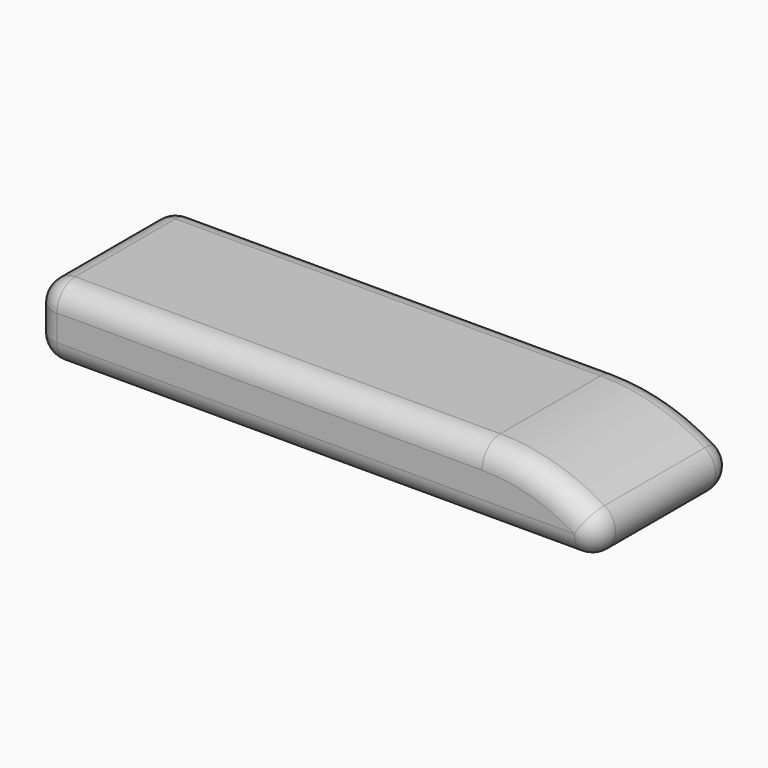
from build123d import *

# Parameters (mm, degrees)
F1_DEPTH     = 38.1
F2_R         = 5.08
F3_F1_R      = 5.08
F3_T2_DEPTH  = 94.7599984092
F3_T4_DEPTH  = 115.3407412507
F3_S8_W      = 5.1816
F3_S8_H      = 5.1816
F3_T9_DEPTH  = 5.1816
F3_S14_W     = 5.1816
F3_S14_H     = 5.1816
F3_T15_DEPTH = 5.1816
F3_T19_ANGLE = 31.4774656297
F3_T21_ANGLE = 148.5225343703
F3_T22_DEPTH = 94.7599984092
F3_T24_DEPTH = 115.3407412507
F3_S28_W     = 5.1816
F3_S28_H     = 5.1816
F3_T29_DEPTH = 5.1816
F3_S34_W     = 5.1816
F3_S34_H     = 5.1816
F3_T35_DEPTH = 5.1816
F3_T39_ANGLE = 31.4774656297
F3_T41_ANGLE = 148.5225343703


# Not quite as in the source:
# - a fillet or chamfer that OpenCascade refuses, or shapes differently, is made with other operations: its cross-section is extruded or revolved along the edge and cut away or added


with BuildPart() as f1:
    # F0 (on Front) → F1 (new body)
    with BuildSketch(Plane.XZ):
        with BuildLine():
            Line((9.9600013345, 7.7700004913), (-89.8799970746, 7.7700004913))
            Line((-89.8799970746, 7.7700004913), (-89.8799970746, -8.1900004297))
            Line((-89.8799970746, -8.1900004297), (44.0999977291, -8.1900004297))
            ThreePointArc((44.0999977291, -8.1900004297), (28.8031763803, 3.5829980082), (9.9600013345, 7.7700004913))
        make_face()
    extrude(amount=F1_DEPTH)

    # F2
    f2_edges = [f1.edges().sort_by_distance(p)[0] for p in [
        (-89.879997, -19.05, -8.19),
        (-89.879997, 0, -0.21),
        (-89.879997, -19.05, 7.77),
        (-89.879997, -38.1, -0.21),
    ]]
    fillet(f2_edges, radius=F2_R)

    # F3: fillet of radius 5.08 on 12 edges, made by hand

    # F3_f1
    f3_f1_edges = [f1.edges().sort_by_distance(p)[0] for p in [
        (44.0999977291, -19.05, -8.1900004297),
    ]]
    fillet(f3_f1_edges, radius=F3_F1_R)

    # F3_s3 → F3_t2 (cut)
    with BuildSketch(Plane.YZ.offset(-84.7999970746)):
        with BuildLine():
            ThreePointArc((0, 2.6900004913), (-1.4878975516, 6.2821029397), (-5.08, 7.7700004913))
            Line((-5.08, 7.7700004913), (-5.08, 7.8716004913))
            Line((-5.08, 7.8716004913), (0.1016, 7.8716004913))
            Line((0.1016, 7.8716004913), (0.1016, 2.6900004913))
            Line((0.1016, 2.6900004913), (0, 2.6900004913))
        make_face()
    extrude(amount=F3_T2_DEPTH, mode=Mode.SUBTRACT)

    # F3_s5 → F3_t4 (cut)
    with BuildSketch(Plane.YZ.offset(-84.7999970746)):
        with BuildLine():
            ThreePointArc((0, -3.1100004297), (-1.4878975516, -6.7021028782), (-5.08, -8.1900004297))
            Line((-5.08, -8.1900004297), (-5.08, -8.2916004297))
            Line((-5.08, -8.2916004297), (0.1016, -8.2916004297))
            Line((0.1016, -8.2916004297), (0.1016, -3.1100004297))
            Line((0.1016, -3.1100004297), (0, -3.1100004297))
        make_face()
    extrude(amount=F3_T4_DEPTH, mode=Mode.SUBTRACT)


with BuildPart() as f3_tool7:
    # F3_s8 → F3_t9 (new body)
    with BuildSketch(Plane.XZ.offset(5.08)):
        with Locations((-87.3907970746, 5.2808004913)):
            Rectangle(F3_S8_W, F3_S8_H)
    extrude(amount=-F3_T9_DEPTH)

    # F3_s10 → F3_t11 (revolve, cut)
    with BuildSketch(Plane(origin=(-84.7999970746, -5.08, 2.6900004913), x_dir=(0.7071067812, 0, -0.7071067812), z_dir=(0.7071067812, 0, 0.7071067812))):
        with BuildLine():
            ThreePointArc((0, -5.08), (5.08, 0), (0, 5.08))
            Line((0, 5.08), (0, -5.08))
        make_face()
    revolve(axis=Axis((-84.7999970746, -5.08, 2.6900004913), (0, 1, 0)), mode=Mode.SUBTRACT)


with BuildPart() as f1_1:
    add(f1.part)

    # F3_t6: cut F3_tool7
    add(f3_tool7.part, mode=Mode.SUBTRACT)


with BuildPart() as f3_tool13:
    # F3_s14 → F3_t15 (new body)
    with BuildSketch(Plane.XZ.offset(5.08)):
        with Locations((-87.3907970746, -5.7008004297)):
            Rectangle(F3_S14_W, F3_S14_H)
    extrude(amount=-F3_T15_DEPTH)

    # F3_s16 → F3_t17 (revolve, cut)
    with BuildSketch(Plane(origin=(-84.7999970746, -5.08, -3.1100004297), x_dir=(0.7071067812, 0, 0.7071067812), z_dir=(-0.7071067812, 0, 0.7071067812))):
        with BuildLine():
            ThreePointArc((0, -5.08), (5.08, 0), (0, 5.08))
            Line((0, 5.08), (0, -5.08))
        make_face()
    revolve(axis=Axis((-84.7999970746, -5.08, -3.1100004297), (0, 1, 0)), mode=Mode.SUBTRACT)


with BuildPart() as f1_2:
    add(f1_1.part)

    # F3_t12: cut F3_tool13
    add(f3_tool13.part, mode=Mode.SUBTRACT)

    # F3_s18 → F3_t19 (revolve, cut)
    with BuildSketch(Plane(origin=(23.5986358548, 0, -14.4484990421), x_dir=(0, 1, 0), z_dir=(0.8528455965, 0, -0.5221631818))):
        with BuildLine():
            ThreePointArc((0, 13.2949019826), (-1.4878975516, 16.887004431), (-5.08, 18.3749019826))
            Line((-5.08, 18.3749019826), (-5.08, 18.4765019826))
            Line((-5.08, 18.4765019826), (0.1016, 18.4765019826))
            Line((0.1016, 18.4765019826), (0.1016, 13.2949019826))
            Line((0.1016, 13.2949019826), (0, 13.2949019826))
        make_face()
    revolve(axis=Axis((9.9600013345, 0, -36.7243886458), (0, -1, 0)), revolution_arc=F3_T19_ANGLE, mode=Mode.SUBTRACT)

    # F3_s20 → F3_t21 (revolve, cut)
    with BuildSketch(Plane(origin=(23.5986358548, 0, -14.4484990421), x_dir=(0, 1, 0), z_dir=(-0.8528455965, 0, 0.5221631818))):
        with BuildLine():
            ThreePointArc((0, -13.2949019826), (-1.4878975516, -16.887004431), (-5.08, -18.3749019826))
            Line((-5.08, -18.3749019826), (-5.08, -18.4765019826))
            Line((-5.08, -18.4765019826), (0.1016, -18.4765019826))
            Line((0.1016, -18.4765019826), (0.1016, -13.2949019826))
            Line((0.1016, -13.2949019826), (0, -13.2949019826))
        make_face()
    revolve(axis=Axis((30.5407441761, 0, -3.1100004297), (0, 1, 0)), revolution_arc=F3_T21_ANGLE, mode=Mode.SUBTRACT)

    # F3_s23 → F3_t22 (cut)
    with BuildSketch(Plane.YZ.offset(-84.7999970746)):
        with BuildLine():
            ThreePointArc((-33.02, 7.7700004913), (-36.6121024484, 6.2821029397), (-38.1, 2.6900004913))
            Line((-38.1, 2.6900004913), (-38.2016, 2.6900004913))
            Line((-38.2016, 2.6900004913), (-38.2016, 7.8716004913))
            Line((-38.2016, 7.8716004913), (-33.02, 7.8716004913))
            Line((-33.02, 7.8716004913), (-33.02, 7.7700004913))
        make_face()
    extrude(amount=F3_T22_DEPTH, mode=Mode.SUBTRACT)

    # F3_s25 → F3_t24 (cut)
    with BuildSketch(Plane.YZ.offset(-84.7999970746)):
        with BuildLine():
            ThreePointArc((-33.02, -8.1900004297), (-36.6121024484, -6.7021028782), (-38.1, -3.1100004297))
            Line((-38.1, -3.1100004297), (-38.2016, -3.1100004297))
            Line((-38.2016, -3.1100004297), (-38.2016, -8.2916004297))
            Line((-38.2016, -8.2916004297), (-33.02, -8.2916004297))
            Line((-33.02, -8.2916004297), (-33.02, -8.1900004297))
        make_face()
    extrude(amount=F3_T24_DEPTH, mode=Mode.SUBTRACT)


with BuildPart() as f3_tool27:
    # F3_s28 → F3_t29 (new body)
    with BuildSketch(Plane.XY.offset(2.6900004913)):
        with Locations((-87.3907970746, -35.6108)):
            Rectangle(F3_S28_W, F3_S28_H)
    extrude(amount=F3_T29_DEPTH)

    # F3_s30 → F3_t31 (revolve, cut)
    with BuildSketch(Plane(origin=(-84.7999970746, -33.02, 2.6900004913), x_dir=(0.7071067812, 0.7071067812, 0), z_dir=(0.7071067812, -0.7071067812, 0))):
        with BuildLine():
            ThreePointArc((0, -5.08), (5.08, 0), (0, 5.08))
            Line((0, 5.08), (0, -5.08))
        make_face()
    revolve(axis=Axis((-84.7999970746, -33.02, 2.6900004913), (0, 0, 1)), mode=Mode.SUBTRACT)


with BuildPart() as f1_3:
    add(f1_2.part)

    # F3_t26: cut F3_tool27
    add(f3_tool27.part, mode=Mode.SUBTRACT)


with BuildPart() as f3_tool33:
    # F3_s34 → F3_t35 (new body)
    with BuildSketch(Plane.XY.offset(-3.1100004297)):
        with Locations((-87.3907970746, -35.6108)):
            Rectangle(F3_S34_W, F3_S34_H)
    extrude(amount=-F3_T35_DEPTH)

    # F3_s36 → F3_t37 (revolve, cut)
    with BuildSketch(Plane(origin=(-84.7999970746, -33.02, -3.1100004297), x_dir=(0.7071067812, 0.7071067812, 0), z_dir=(-0.7071067812, 0.7071067812, 0))):
        with BuildLine():
            ThreePointArc((0, -5.08), (5.08, 0), (0, 5.08))
            Line((0, 5.08), (0, -5.08))
        make_face()
    revolve(axis=Axis((-84.7999970746, -33.02, -3.1100004297), (0, 0, -1)), mode=Mode.SUBTRACT)


with BuildPart() as f1_4:
    add(f1_3.part)

    # F3_t32: cut F3_tool33
    add(f3_tool33.part, mode=Mode.SUBTRACT)

    # F3_s38 → F3_t39 (revolve, cut)
    with BuildSketch(Plane(origin=(23.5986358548, 0, -14.4484990421), x_dir=(0, 1, 0), z_dir=(0.8528455965, 0, -0.5221631818))):
        with BuildLine():
            ThreePointArc((-33.02, 18.3749019826), (-36.6121024484, 16.887004431), (-38.1, 13.2949019826))
            Line((-38.1, 13.2949019826), (-38.2016, 13.2949019826))
            Line((-38.2016, 13.2949019826), (-38.2016, 18.4765019826))
            Line((-38.2016, 18.4765019826), (-33.02, 18.4765019826))
            Line((-33.02, 18.4765019826), (-33.02, 18.3749019826))
        make_face()
    revolve(axis=Axis((9.9600013345, -38.1, -36.7243886458), (0, -1, 0)), revolution_arc=F3_T39_ANGLE, mode=Mode.SUBTRACT)

    # F3_s40 → F3_t41 (revolve, cut)
    with BuildSketch(Plane(origin=(23.5986358548, 0, -14.4484990421), x_dir=(0, 1, 0), z_dir=(-0.8528455965, 0, 0.5221631818))):
        with BuildLine():
            ThreePointArc((-33.02, -18.3749019826), (-36.6121024484, -16.887004431), (-38.1, -13.2949019826))
            Line((-38.1, -13.2949019826), (-38.2016, -13.2949019826))
            Line((-38.2016, -13.2949019826), (-38.2016, -18.4765019826))
            Line((-38.2016, -18.4765019826), (-33.02, -18.4765019826))
            Line((-33.02, -18.4765019826), (-33.02, -18.3749019826))
        make_face()
    revolve(axis=Axis((30.5407441761, -38.1, -3.1100004297), (0, 1, 0)), revolution_arc=F3_T41_ANGLE, mode=Mode.SUBTRACT)


solid = f1_4.part
